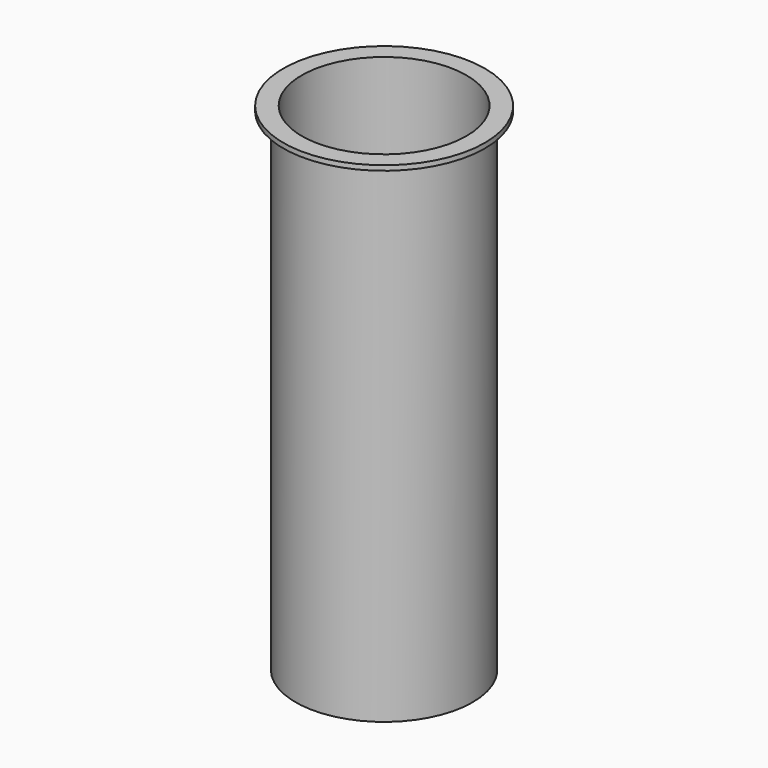
from build123d import *

# Parameters (mm, degrees)
F0_R     = 41
F0_R_2   = 36
F1_DEPTH = 2
F2_DEPTH = 200
F3_T     = 2.5
F5_R     = 23.5
F6_DEPTH = 25
F7_SIZE  = 9.99999


# Not quite as in the source:
# - a fillet or chamfer is up to 0.001 mm smaller than in the source, because OpenCascade refuses the exact size
# - a shell that OpenCascade refuses in one call is made with other operations: the cavity is built on its own and cut out


with BuildPart() as f1:
    # F0 (on Top) → F1 (new body)
    with BuildSketch(Plane.XY):
        Circle(F0_R)
        Circle(F0_R_2, mode=Mode.SUBTRACT)
        Circle(F0_R_2)
    extrude(amount=F1_DEPTH)

    # F0 (on Top) → F2 (join)
    with BuildSketch(Plane.XY):
        Circle(F0_R_2)
    extrude(amount=-F2_DEPTH)

    # F3: shell of thickness 2.5, made by hand


with BuildPart() as f3_core1:
    # F3_t2: copy of F1
    add(f1.part)

    # the walls: a layer under each face that stays
    f3_faces = [f3_core1.faces().sort_by_distance(p)[0] for p in [
        (-41, 0, 1),
        (-27.3333333333, -27.3333333333, 0),
        (-36, 0, -100),
        (0, 0, -200),
    ]]
    thicken(f3_faces, amount=-F3_T, mode=Mode.SUBTRACT)

    # F3_s3 → F3_t4 (revolve, cut)
    with BuildSketch(Plane.XZ):
        Polygon((36.025, -0.025), (36, 2.5), (33.5, 2.5), (33.5, 0), align=None)
    revolve(axis=Axis((0, 0, 0), (0, 0, 1)), mode=Mode.SUBTRACT)


with BuildPart() as f1_1:
    add(f1.part)

    # what is left inside the walls is the cavity
    f3_cavity = [f3_core1.part.solids().sort_by_distance(p)[0] for p in [
        (-33.475, 0, -64.5),
    ]]
    add(f3_cavity, mode=Mode.SUBTRACT)

    # F5 (on offset) → F6 (cut)
    with BuildSketch(Plane(origin=(0, 0, -200), x_dir=(1, 0, 0), z_dir=(0, 0, -1))):
        Circle(F5_R)
    extrude(amount=-F6_DEPTH, mode=Mode.SUBTRACT)

    # F7 (size 10 in the source; OpenCascade refuses exactly that, so slightly less here)
    f7_edges = [f1_1.edges().sort_by_distance(p)[0] for p in [
        (33.5, 0, -97.75),
        (-33.5, 0, -197.5),
    ]]
    chamfer(f7_edges, length=F7_SIZE)


solid = f1_1.part
